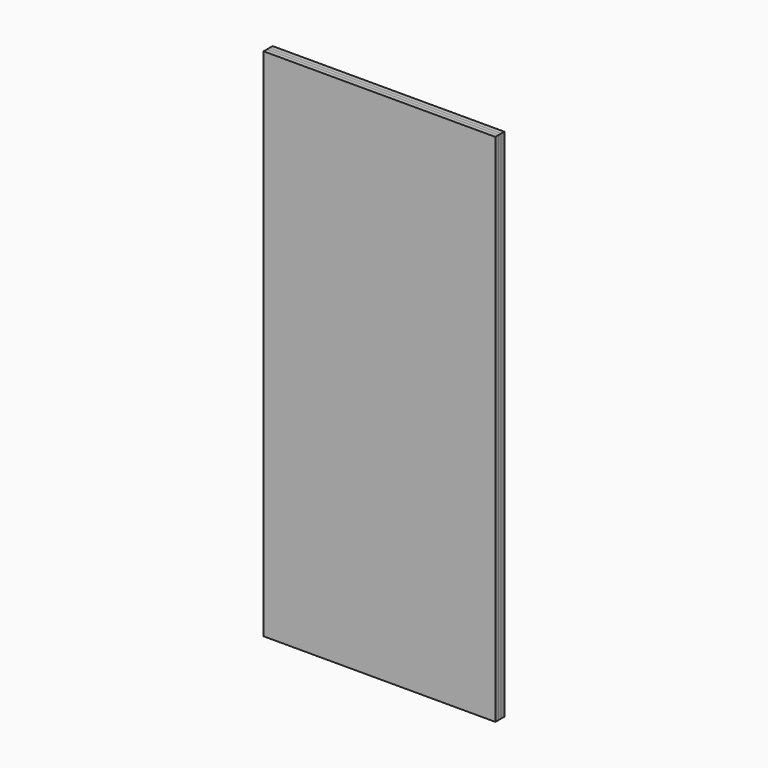
from build123d import *

# Parameters (mm, degrees)
F0_W     = 914.4
F0_H     = 2032
F1_DEPTH = 22.225
F2_T     = -6.35
F3_W     = 914.4
F3_H     = 2032
F4_DEPTH = 6.35


# Not quite as in the source:
# - the dataset's text gives a spline's control points without its knots; the knots are read off the source's solid
# - a feature names something its author has since deleted; it is built from what else it names


with BuildPart() as f1:
    # F0 (on Front) → F1 (new body, symmetric)
    with BuildSketch(Plane.XZ):
        Rectangle(F0_W, F0_H)
    extrude(amount=F1_DEPTH, both=True)

    # F2 (hollow: no face is removed)
    offset(amount=F2_T, mode=Mode.SUBTRACT)


with BuildPart() as f4:
    # F3 (on Front) → F4 (new body, symmetric)
    with BuildSketch(Plane.XZ):
        Rectangle(F3_W, F3_H)
        with BuildLine():
            add(Edge.make_bspline(
                [(-102.788878744, 53.0522555544), (-115.0796561664, 57.7747130109), (-172.109902554, 75.8931860417), (-272.4486443535, 70.1170066616), (-353.7320815536, 40.4856256956), (-402.3453308508, -20.8974867371), (-411.9104648371, -45.9242845247), (-415.8637821674, -56.2679842114)],
                knots=[0.1925412434, 0.1925412434, 0.1925412434, 0.1925412434, 0.2598556278, 0.5007810461, 0.6941216382, 0.8735789556, 1, 1, 1, 1], degree=3))
            ThreePointArc((-102.788878744, 53.0522555544), (27.297096775, 112.4053553907), (115.6723623553, 0))
            ThreePointArc((115.6723623553, 0), (-8.3781922539, -115.368545572), (-114.4586911894, 16.7123733823))
            add(Edge.make_bspline(
                [(-114.4586911894, 16.7123733823), (-119.373915653, 18.6409773824), (-126.780010707, 21.3246804139), (-135.3769480544, 24.0011548026), (-140.3568205391, 25.4145011425), (-144.0830186716, 26.4018437315), (-147.1822873269, 27.1632650826), (-149.6569220432, 27.7345753336), (-153.3861427683, 28.5587482576), (-159.0370105211, 29.6716080851), (-166.6748632527, 30.8983238142), (-174.3948906026, 31.8744426293), (-182.175713824, 32.607269398), (-192.6017748616, 33.2707129632), (-205.6752257784, 33.5333589987), (-221.2462439818, 33.019172763), (-233.9701770212, 31.9719071287), (-243.904748781, 30.8102997522), (-251.2096448082, 29.7898690479), (-257.1560475615, 28.8258650751), (-261.8154455178, 27.9934473686), (-265.2608722389, 27.33969481), (-268.6427806681, 26.6605890428), (-273.039065215, 25.726133421), (-278.3374380434, 24.4991846311), (-284.3834831204, 22.9279699464), (-292.0432019853, 20.6943122087), (-300.8925913227, 17.6307385606), (-308.8851535917, 14.1698326237), (-314.8583988735, 11.1266815586), (-319.1554720592, 8.6930736846), (-323.298239195, 6.0910038781), (-326.3105701104, 3.9977373945), (-328.2890021767, 2.5346327242), (-329.5984230491, 1.5422377588), (-331.2419023871, 0.2509479554), (-333.2206947963, -1.3764025092), (-335.8596426843, -3.6424838525), (-339.1459948656, -6.6423529507), (-343.0294781647, -10.4641063031), (-346.8163532922, -14.459813445), (-350.4730691017, -18.5798240363), (-353.9684413043, -22.7729503539), (-357.273045034, -26.9863828828), (-360.3585883118, -31.1651712353), (-363.1976042652, -35.2518241058), (-365.3345588114, -38.5282614985), (-366.8937992739, -41.039502175), (-367.9816193163, -42.8537563567), (-368.9967401066, -44.6097462535), (-370.267963964, -46.89150151), (-371.7173740536, -49.6457172315), (-373.2876715658, -52.858174126), (-375.2232016159, -57.1070610359), (-377.4658419186, -62.5281453327), (-379.2973206299, -67.3131809286), (-380.2745405787, -69.8700385835)],
                knots=[0.1884362819, 0.1884362819, 0.1884362819, 0.1884362819, 0.21875, 0.234375, 0.2421875, 0.25, 0.2578125, 0.26171875, 0.265625, 0.28125, 0.296875, 0.3125, 0.328125, 0.34375, 0.375, 0.40625, 0.4375, 0.453125, 0.46875, 0.484375, 0.4921875, 0.5, 0.5078125, 0.515625, 0.53125, 0.546875, 0.5625, 0.59375, 0.625, 0.640625, 0.65625, 0.671875, 0.6875, 0.69140625, 0.6953125, 0.703125, 0.7109375, 0.71875, 0.734375, 0.75, 0.765625, 0.78125, 0.796875, 0.8125, 0.828125, 0.84375, 0.859375, 0.8671875, 0.875, 0.8828125, 0.890625, 0.90625, 0.921875, 0.9375, 0.96875, 1, 1, 1, 1], degree=3))
            Line((-380.2745405787, -69.8700385835), (-392.1376211083, -65.3360204595))
            Line((-392.1376211083, -65.3360204595), (-404.0007016379, -60.8020023355))
            Line((-404.0007016379, -60.8020023355), (-415.8637821674, -56.2679842114))
        make_face(mode=Mode.SUBTRACT)
    extrude(amount=F4_DEPTH, both=True)


with BuildPart() as f4b:
    # F3 (on Front) → F4, piece 2 (new body, symmetric)
    with BuildSketch(Plane.XZ):
        with BuildLine():
            Line((37.3285076505, 64.6548718214), (-37.3285076505, 64.6548718214))
            Line((-37.3285076505, 64.6548718214), (-56.3298401221, 31.7435985691))
            add(Edge.make_bspline(
                [(0, 0), (-18.7011235658, 10.9343625548), (-37.4022471317, 21.8687251095), (-56.3298401221, 31.7435985691)],
                knots=[0, 0, 0, 0, 0.1064783731, 0.1064783731, 0.1064783731, 0.1064783731], degree=3))
            Line((0, 0), (-6.4102574675, -10.9635121745))
            Line((-6.4102574675, -10.9635121745), (-12.8205149351, -21.9270243489))
            Line((-12.8205149351, -21.9270243489), (-19.2307724026, -32.8905365234))
            add(Edge.make_bspline(
                [(-19.2307724026, -32.8905365234), (-30.2078392868, -26.4723537507), (-46.4073877333, -17.00410068), (-64.2129954804, -7.1787118869), (-71.3710947537, -3.3861690523), (-73.2781581831, -2.3882505846)],
                knots=[0, 0, 0, 0, 0.0625, 0.09375, 0.1051349345, 0.1051349345, 0.1051349345, 0.1051349345], degree=3))
            Line((-73.2781581831, -2.3882505846), (-37.3285076505, -64.6548718214))
            Line((-37.3285076505, -64.6548718214), (37.3285076505, -64.6548718214))
            Line((37.3285076505, -64.6548718214), (74.657015301, 0))
            Line((74.657015301, 0), (37.3285076505, 64.6548718214))
        make_face()
    extrude(amount=F4_DEPTH, both=True)


solid = Compound([f1.part, f4.part, f4b.part])
